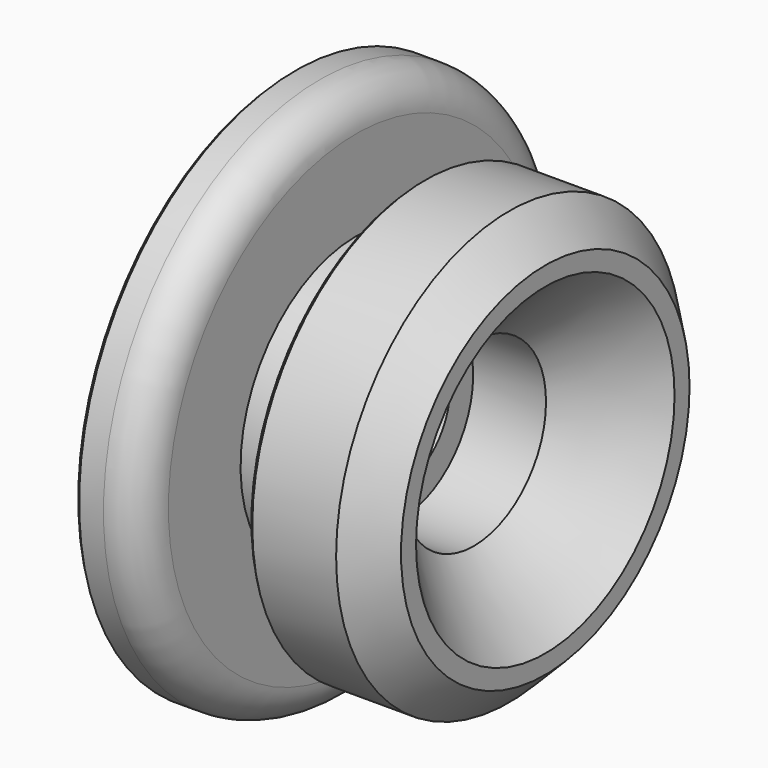
from build123d import *

# Parameters (mm, degrees)
F0_R           = 15
F1_DEPTH       = 3.6
F2_R           = 12
F3_DEPTH       = 10.5
F5_D           = 6.8
F5_CSINK_D     = 17.92
F5_CSINK_ANGLE = 90
F6_W           = 3.6
F6_H           = 5
F8_SIZE        = 0.25
F9_R           = 2
F10_SIZE       = 2
F11_R          = 5
F12_DEPTH      = 8


with BuildPart() as f1:
    # F0 (on Right) → F1 (new body)
    with BuildSketch(Plane.YZ):
        Circle(F0_R)
    extrude(amount=F1_DEPTH)

    # F2 (on face) → F3 (join)
    with BuildSketch(Plane.YZ.offset(3.6)):
        Circle(F2_R)
    extrude(amount=F3_DEPTH)

    # F5 (through all)
    with Locations(Plane.YZ.offset(14.1)):
        with Locations((0, 0)):
            CounterSinkHole(F5_D / 2, F5_CSINK_D / 2, counter_sink_angle=F5_CSINK_ANGLE)

    # F6 (on Front) → F7 (revolve, cut)
    with BuildSketch(Plane.XZ):
        with Locations((5.4, 10.5)):
            Rectangle(F6_W, F6_H)
    revolve(axis=Axis((8.5571676374, 0, 0), (1, 0, 0)), mode=Mode.SUBTRACT)

    # F8
    f8_edges = [f1.edges().sort_by_distance(p)[0] for p in [
        (0, -15, 0),
        (7.2, -12, 0),
    ]]
    chamfer(f8_edges, length=F8_SIZE)

    # F9
    f9_edges = [f1.edges().sort_by_distance(p)[0] for p in [
        (3.6, -15, 0),
    ]]
    fillet(f9_edges, radius=F9_R)

    # F10
    f10_edges = [f1.edges().sort_by_distance(p)[0] for p in [
        (14.1, -12, 0),
    ]]
    chamfer(f10_edges, length=F10_SIZE)

    # F11 (on face) → F12 (cut)
    with BuildSketch(Plane.YZ.offset(14.1)):
        Circle(F11_R)
    extrude(amount=-F12_DEPTH, mode=Mode.SUBTRACT)


solid = f1.part
